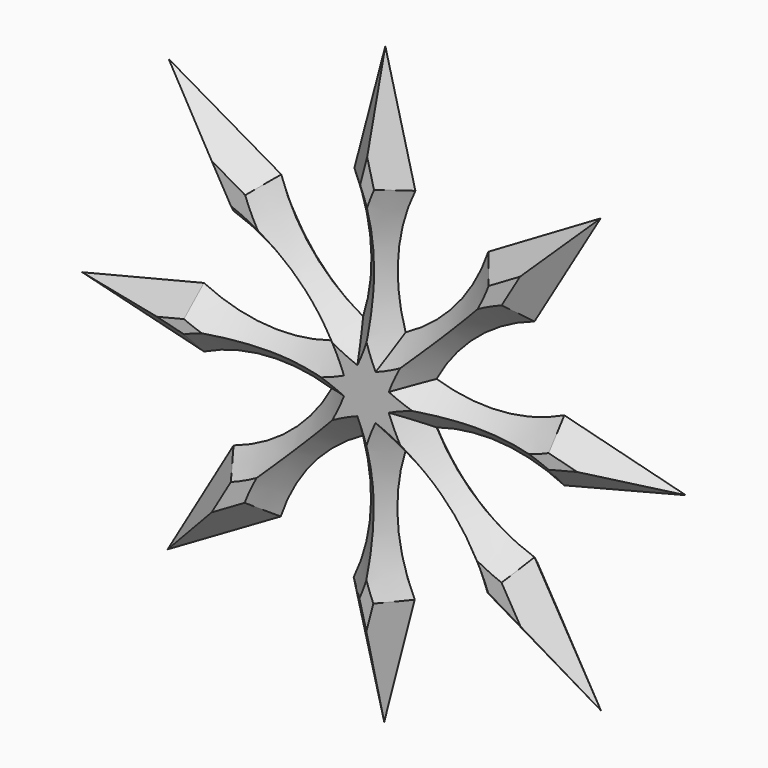
from build123d import *

# Parameters (mm, degrees)
F1_DEPTH      = 3.81
F2_T3_ANGLE   = 94.2071978341
F2_S4_R       = 28.267340588
F2_T5_DEPTH   = 27
F2_T8_DEPTH   = 53.0413211694
F2_T11_DEPTH  = 53.0413211694
F2_T14_ANGLE  = 94.2071978341
F2_S15_R      = 28.267340588
F2_T16_DEPTH  = 27
F2_T19_ANGLE  = 94.2071978341
F2_S20_R      = 28.267340588
F2_T21_DEPTH  = 26
F2_T24_DEPTH  = 53.791822705
F2_T27_DEPTH  = 53.791822705
F2_T30_ANGLE  = 94.2071978341
F2_S31_R      = 28.267340588
F2_T32_DEPTH  = 26
F2_T35_ANGLE  = 94.2071978341
F2_S36_R      = 28.267340588
F2_T37_DEPTH  = 27
F2_T40_DEPTH  = 52.2617558208
F2_T43_DEPTH  = 52.2617558208
F2_T46_ANGLE  = 94.2071978341
F2_S47_R      = 28.267340588
F2_T48_DEPTH  = 27
F2_T51_ANGLE  = 94.2071978341
F2_S52_R      = 28.267340588
F2_T53_DEPTH  = 26
F2_T56_DEPTH  = 53.6108831217
F2_T59_DEPTH  = 53.6108831217
F2_T62_ANGLE  = 94.2071978341
F2_S63_R      = 28.267340588
F2_T64_DEPTH  = 26
F2_T67_ANGLE  = 94.2071978341
F2_S68_R      = 28.267340588
F2_T69_DEPTH  = 27
F2_T72_DEPTH  = 53.1727745631
F2_T75_DEPTH  = 53.1727745631
F2_T78_ANGLE  = 94.2071978341
F2_S79_R      = 28.267340588
F2_T80_DEPTH  = 27
F2_T83_ANGLE  = 94.2071978341
F2_S84_R      = 28.267340588
F2_T85_DEPTH  = 26
F2_T88_DEPTH  = 53.7976919269
F2_T91_DEPTH  = 53.7976919269
F2_T94_ANGLE  = 94.2071978341
F2_S95_R      = 28.267340588
F2_T96_DEPTH  = 26
F2_T99_ANGLE  = 94.2071978341
F2_S100_R     = 28.267340588
F2_T101_DEPTH = 27
F2_T104_DEPTH = 52.2617558208
F2_T107_DEPTH = 52.2617558208
F2_T110_ANGLE = 94.2071978341
F2_S111_R     = 28.267340588
F2_T112_DEPTH = 27
F2_T115_ANGLE = 94.2071978341
F2_S116_R     = 28.267340588
F2_T117_DEPTH = 26
F2_T120_DEPTH = 53.9557904265
F2_T123_DEPTH = 53.9557904265
F2_T126_ANGLE = 94.2071978341
F2_S127_R     = 28.267340588
F2_T128_DEPTH = 26
F2_T132_ANGLE = 94.2071978341
F2_S133_R     = 28.267340588
F2_T134_DEPTH = 27
F2_T138_ANGLE = 94.2071978341
F2_S139_R     = 28.267340588
F2_T140_DEPTH = 26
F2_T146_ANGLE = 94.2071978341
F2_S147_R     = 28.267340588
F2_T148_DEPTH = 27
F2_T152_ANGLE = 94.2071978341
F2_S153_R     = 28.267340588
F2_T154_DEPTH = 26
F2_T160_ANGLE = 94.2071978341
F2_S161_R     = 28.267340588
F2_T162_DEPTH = 26
F2_T166_ANGLE = 94.2071978341
F2_S167_R     = 28.267340588
F2_T168_DEPTH = 27
F2_T174_ANGLE = 94.2071978341
F2_S175_R     = 28.267340588
F2_T176_DEPTH = 27
F2_T180_ANGLE = 94.2071978341
F2_S181_R     = 28.267340588
F2_T182_DEPTH = 26
F2_T188_ANGLE = 94.2071978341
F2_S189_R     = 28.267340588
F2_T190_DEPTH = 26
F2_T194_ANGLE = 94.2071978341
F2_S195_R     = 28.267340588
F2_T196_DEPTH = 27
F2_T202_ANGLE = 94.2071978341
F2_S203_R     = 28.267340588
F2_T204_DEPTH = 27
F2_T208_ANGLE = 94.2071978341
F2_S209_R     = 28.267340588
F2_T210_DEPTH = 26
F2_T216_ANGLE = 94.2071978341
F2_S217_R     = 28.267340588
F2_T218_DEPTH = 26
F2_T222_ANGLE = 94.2071978341
F2_S223_R     = 28.267340588
F2_T224_DEPTH = 27
F2_T230_ANGLE = 94.2071978341
F2_S231_R     = 28.267340588
F2_T232_DEPTH = 27
F2_T236_ANGLE = 94.2071978341
F2_S237_R     = 28.267340588
F2_T238_DEPTH = 26


# Not quite as in the source:
# - a fillet or chamfer that OpenCascade refuses, or shapes differently, is made with other operations: its cross-section is extruded or revolved along the edge and cut away or added


with BuildPart() as f1:
    # F0 (on Front) → F1 (new body)
    with BuildSketch(Plane.XZ):
        with BuildLine():
            Line((6.679601036, 30.6390393525), (0.209001727, 55.9587727979))
            Line((0.209001727, 55.9587727979), (-6.4505489481, 30.6880794563))
            ThreePointArc((-6.4505489481, 30.6880794563), (-3.6066981966, 20.9770503759), (-4.3651827706, 10.8866453272))
            ThreePointArc((-4.3651827706, 10.8866453272), (-11.8846232574, 17.6578776863), (-16.5375233069, 26.6435381532))
            Line((-16.5375233069, 26.6435381532), (-40.327632255, 40.403012619))
            Line((-40.327632255, 40.403012619), (-26.6126086657, 16.5872499967))
            ThreePointArc((-26.6126086657, 16.5872499967), (-17.6356529341, 11.9175777716), (-10.8784745754, 4.3855054456))
            ThreePointArc((-10.8784745754, 4.3855054456), (-20.970278463, 3.6458655403), (-30.6759798559, 6.5078462128))
            Line((-30.6759798559, 6.5078462128), (-56.9257720003, 0))
            Line((-56.9257720003, 0), (-30.6759798559, -6.5078462128))
            ThreePointArc((-30.6759798559, -6.5078462128), (-20.970278463, -3.6458655403), (-10.8784745754, -4.3855054456))
            ThreePointArc((-10.8784745754, -4.3855054456), (-17.6356529341, -11.9175777716), (-26.6126086657, -16.5872499967))
            Line((-26.6126086657, -16.5872499967), (-40.5599377533, -40.4842646123))
            Line((-40.5599377533, -40.4842646123), (-16.6369188404, -26.58158637))
            ThreePointArc((-16.6369188404, -26.58158637), (-11.9504907247, -17.6133666797), (-4.4058128267, -10.8702658862))
            ThreePointArc((-4.4058128267, -10.8702658862), (-3.6850201695, -20.9634334188), (-6.5651207822, -30.6637732767))
            Line((-6.5651207822, -30.6637732767), (0, -55.9591630992))
            Line((0, -55.9591630992), (6.5651207822, -30.6637732767))
            ThreePointArc((6.5651207822, -30.6637732767), (3.6850201695, -20.9634334188), (4.4058128267, -10.8702658862))
            ThreePointArc((4.4058128267, -10.8702658862), (11.9504907247, -17.6133666797), (16.6369188404, -26.58158637))
            Line((16.6369188404, -26.58158637), (40.6195603878, -40.6954864235))
            Line((40.6195603878, -40.6954864235), (26.5504713741, -16.6865296649))
            ThreePointArc((26.5504713741, -16.6865296649), (17.5910190008, -11.9833620019), (10.8620192883, -4.4261048431))
            ThreePointArc((10.8620192883, -4.4261048431), (20.9565152672, -3.7241619477), (30.6514597612, -6.6223724565))
            Line((30.6514597612, -6.6223724565), (56.7369909394, 0))
            Line((56.7369909394, 0), (30.6514597612, 6.6223724565))
            ThreePointArc((30.6514597612, 6.6223724565), (20.9565152672, 3.7241619477), (10.8620192883, 4.4261048431))
            ThreePointArc((10.8620192883, 4.4261048431), (17.5910190008, 11.9833620019), (26.5504713741, 16.6865296649))
            Line((26.5504713741, 16.6865296649), (40.5952992978, 40.5195601823))
            Line((40.5952992978, 40.5195601823), (16.7360822971, 26.5192637868))
            ThreePointArc((16.7360822971, 26.5192637868), (12.0161914886, 17.5686099753), (4.4463814239, 10.8537348104))
            ThreePointArc((4.4463814239, 10.8537348104), (3.7632907382, 20.9495240322), (6.679601036, 30.6390393525))
        make_face()
    extrude(amount=F1_DEPTH)

    # F2: chamfer of 5.08 on 32 edges, made by hand


with BuildPart() as f2_tool1:
    # F2_s2 → F2_t3 (revolve)
    with BuildSketch(Plane(origin=(-5.5052343912, 0, -4.7470845502), x_dir=(0, 1, 0), z_dir=(-0.757328805, 0, -0.6530337519))):
        Polygon((1.27, 7.4792542612), (-3.81, 2.3992542612), (-3.81, 7.4792542612), align=None)
    revolve(axis=Axis((17.838498561, -3.81, -31.8190105099), (0, 1, 0)), revolution_arc=F2_T3_ANGLE)

    # F2_s4 → F2_t5 (intersect, symmetric)
    with BuildSketch(Plane.XZ.offset(1.3)):
        with Locations((34.9970077729, 10.289358954)):
            Circle(F2_S4_R)
    extrude(amount=F2_T5_DEPTH, both=True, mode=Mode.INTERSECT)


with BuildPart() as f2_tool6:
    # F2_s7 → F2_t8 (new body)
    with BuildSketch(Plane(origin=(14.5536608526, 0, 3.6947594478), x_dir=(0, 1, 0), z_dir=(0.9692531432, 0, 0.2460657318))):
        Polygon((1.27, -13.9610291961), (-3.81, -8.8810291961), (-3.81, -13.9610291961), align=None)
    extrude(amount=F2_T8_DEPTH)


with BuildPart() as f2_tool9:
    # F2_s10 → F2_t11 (new body)
    with BuildSketch(Plane(origin=(65.9641281162, 0, -16.7464109574), x_dir=(0, 1, 0), z_dir=(-0.9692531432, 0, 0.2460657318))):
        Polygon((1.27, -13.9610291961), (-3.81, -8.8810291961), (-3.81, -13.9610291961), align=None)
    extrude(amount=F2_T11_DEPTH)


with BuildPart() as f2_tool12:
    # F2_s13 → F2_t14 (revolve)
    with BuildSketch(Plane(origin=(21.55504735, 0, 29.0625266695), x_dir=(0, 1, 0), z_dir=(0.595713721, 0, 0.8031968393))):
        Polygon((1.27, -23.6401451022), (-3.81, -28.7201451022), (-3.81, -23.6401451022), align=None)
    revolve(axis=Axis((17.838498561, -3.81, 31.8190105099), (0, 1, 0)), revolution_arc=F2_T14_ANGLE)

    # F2_s15 → F2_t16 (intersect, symmetric)
    with BuildSketch(Plane.XZ.offset(1.3)):
        with Locations((34.9970077729, -10.289358954)):
            Circle(F2_S15_R)
    extrude(amount=F2_T16_DEPTH, both=True, mode=Mode.INTERSECT)


with BuildPart() as f2_tool17:
    # F2_s18 → F2_t19 (revolve)
    with BuildSketch(Plane(origin=(-0.6195292674, 0, -7.2428310015), x_dir=(0, 1, 0), z_dir=(-0.0852256828, 0, -0.9963616728))):
        Polygon((1.27, 7.4792542612), (-3.81, 2.3992542612), (-3.81, 7.4792542612), align=None)
    revolve(axis=Axis((34.9970077729, -3.81, -10.289358954), (0, 1, 0)), revolution_arc=F2_T19_ANGLE)

    # F2_s20 → F2_t21 (intersect, symmetric)
    with BuildSketch(Plane.XZ.offset(1.3)):
        with Locations((17.838498561, 31.8190105099)):
            Circle(F2_S20_R)
    extrude(amount=F2_T21_DEPTH, both=True, mode=Mode.INTERSECT)


with BuildPart() as f2_tool22:
    # F2_s23 → F2_t24 (new body)
    with BuildSketch(Plane(origin=(7.5097109066, 0, 12.7434220047), x_dir=(0, 1, 0), z_dir=(0.5077020612, 0, 0.8615327139))):
        Polygon((1.27, -14.4023141537), (-3.81, -9.3223141537), (-3.81, -14.4023141537), align=None)
    extrude(amount=F2_T24_DEPTH)


with BuildPart() as f2_tool25:
    # F2_s26 → F2_t27 (new body)
    with BuildSketch(Plane(origin=(59.1517585206, 0, 34.7095276255), x_dir=(0, 1, 0), z_dir=(-0.8624793208, 0, -0.506092305))):
        Polygon((1.27, -14.4023141537), (-3.81, -9.3223141537), (-3.81, -14.4023141537), align=None)
    extrude(amount=F2_T27_DEPTH)


with BuildPart() as f2_tool28:
    # F2_s29 → F2_t30 (revolve)
    with BuildSketch(Plane(origin=(-5.6536224324, 0, 35.7391532646), x_dir=(0, 1, 0), z_dir=(-0.1562483441, 0, 0.9877178013))):
        Polygon((1.27, -23.6401451022), (-3.81, -28.7201451022), (-3.81, -23.6401451022), align=None)
    revolve(axis=Axis((-10.2239857837, -3.81, 35.0161616319), (0, 1, 0)), revolution_arc=F2_T30_ANGLE)

    # F2_s31 → F2_t32 (intersect, symmetric)
    with BuildSketch(Plane.XZ.offset(1.3)):
        with Locations((31.8522675655, 17.7790469844)):
            Circle(F2_S31_R)
    extrude(amount=F2_T32_DEPTH, both=True, mode=Mode.INTERSECT)


with BuildPart() as f2_tool33:
    # F2_s34 → F2_t35 (revolve)
    with BuildSketch(Plane(origin=(4.7367955124, 0, -5.5140897439), x_dir=(0, 1, 0), z_dir=(0.6516183381, 0, -0.7585469936))):
        Polygon((1.27, 7.4792542612), (-3.81, 2.3992542612), (-3.81, 7.4792542612), align=None)
    revolve(axis=Axis((31.8522675655, -3.81, 17.7790469844), (0, 1, 0)), revolution_arc=F2_T35_ANGLE)

    # F2_s36 → F2_t37 (intersect, symmetric)
    with BuildSketch(Plane.XZ.offset(1.3)):
        with Locations((-10.2239857837, 35.0161616319)):
            Circle(F2_S36_R)
    extrude(amount=F2_T37_DEPTH, both=True, mode=Mode.INTERSECT)


with BuildPart() as f2_tool38:
    # F2_s39 → F2_t40 (new body)
    with BuildSketch(Plane(origin=(-3.7058079888, 0, 14.5009860748), x_dir=(0, 1, 0), z_dir=(-0.2475982949, 0, 0.9688627789))):
        Polygon((1.27, -14.0577907221), (-3.81, -8.9777907221), (-3.81, -14.0577907221), align=None)
    extrude(amount=F2_T40_DEPTH)


with BuildPart() as f2_tool41:
    # F2_s42 → F2_t43 (new body)
    with BuildSketch(Plane(origin=(17.1318103034, 0, 65.0092995281), x_dir=(0, 1, 0), z_dir=(-0.2548285426, 0, -0.9669862532))):
        Polygon((1.27, -14.0577907221), (-3.81, -8.9777907221), (-3.81, -14.0577907221), align=None)
    extrude(amount=F2_T43_DEPTH)


with BuildPart() as f2_tool44:
    # F2_s45 → F2_t46 (revolve)
    with BuildSketch(Plane(origin=(-28.9413121051, 0, 21.7175269383), x_dir=(0, 1, 0), z_dir=(-0.7998468499, 0, 0.6002041458))):
        Polygon((1.27, -23.6401451022), (-3.81, -28.7201451022), (-3.81, -23.6401451022), align=None)
    revolve(axis=Axis((-31.718574019, -3.81, 18.0164792049), (0, 1, 0)), revolution_arc=F2_T46_ANGLE)

    # F2_s47 → F2_t48 (intersect, symmetric)
    with BuildSketch(Plane.XZ.offset(1.3)):
        with Locations((10.4852622562, 34.9388141779)):
            Circle(F2_S47_R)
    extrude(amount=F2_T48_DEPTH, both=True, mode=Mode.INTERSECT)


with BuildPart() as f2_tool49:
    # F2_s50 → F2_t51 (revolve)
    with BuildSketch(Plane(origin=(7.2392465313, 0, -0.660096272), x_dir=(0, 1, 0), z_dir=(0.9958685743, 0, -0.0908062919))):
        Polygon((1.27, 7.4792542612), (-3.81, 2.3992542612), (-3.81, 7.4792542612), align=None)
    revolve(axis=Axis((10.4852622562, -3.81, 34.9388141779), (0, 1, 0)), revolution_arc=F2_T51_ANGLE)

    # F2_s52 → F2_t53 (intersect, symmetric)
    with BuildSketch(Plane.XZ.offset(1.3)):
        with Locations((-31.718574019, 18.0164792049)):
            Circle(F2_S52_R)
    extrude(amount=F2_T53_DEPTH, both=True, mode=Mode.INTERSECT)


with BuildPart() as f2_tool54:
    # F2_s55 → F2_t56 (new body)
    with BuildSketch(Plane(origin=(-12.6304595626, 0, 7.3050731387), x_dir=(0, 1, 0), z_dir=(-0.8656430916, 0, 0.5006616002))):
        Polygon((1.27, -14.7840918558), (-3.81, -9.7040918558), (-3.81, -14.7840918558), align=None)
    extrude(amount=F2_T56_DEPTH)


with BuildPart() as f2_tool57:
    # F2_s58 → F2_t59 (new body)
    with BuildSketch(Plane(origin=(-34.0356728526, 0, 59.1020132098), x_dir=(0, 1, 0), z_dir=(0.4990441804, 0, -0.8665765437))):
        Polygon((1.27, -14.7840918558), (-3.81, -9.7040918558), (-3.81, -14.7840918558), align=None)
    extrude(amount=F2_T59_DEPTH)


with BuildPart() as f2_tool60:
    # F2_s61 → F2_t62 (revolve)
    with BuildSketch(Plane(origin=(-35.7069189472, 0, -5.8537562277), x_dir=(0, 1, 0), z_dir=(-0.9868269461, 0, -0.1617794128))):
        Polygon((1.27, -23.6401451022), (-3.81, -28.7201451022), (-3.81, -23.6401451022), align=None)
    revolve(axis=Axis((-34.9583339784, -3.81, -10.419997418), (0, 1, 0)), revolution_arc=F2_T62_ANGLE)

    # F2_s63 → F2_t64 (intersect, symmetric)
    with BuildSketch(Plane.XZ.offset(1.3)):
        with Locations((-17.9572148782, 31.7521636201)):
            Circle(F2_S63_R)
    extrude(amount=F2_T64_DEPTH, both=True, mode=Mode.INTERSECT)


with BuildPart() as f2_tool65:
    # F2_s66 → F2_t67 (revolve)
    with BuildSketch(Plane(origin=(5.4874661203, 0, 4.7676129256), x_dir=(0, 1, 0), z_dir=(0.7548845088, 0, 0.6558577425))):
        Polygon((1.27, 7.4792542612), (-3.81, 2.3992542612), (-3.81, 7.4792542612), align=None)
    revolve(axis=Axis((-17.9572148782, -3.81, 31.7521636201), (0, 1, 0)), revolution_arc=F2_T67_ANGLE)

    # F2_s68 → F2_t69 (intersect, symmetric)
    with BuildSketch(Plane.XZ.offset(1.3)):
        with Locations((-34.9583339784, -10.419997418)):
            Circle(F2_S68_R)
    extrude(amount=F2_T69_DEPTH, both=True, mode=Mode.INTERSECT)


with BuildPart() as f2_tool70:
    # F2_s71 → F2_t72 (new body)
    with BuildSketch(Plane(origin=(-14.6994140485, 0, -3.6442774678), x_dir=(0, 1, 0), z_dir=(-0.9706156896, 0, -0.2406349584))):
        Polygon((1.27, -13.6983307744), (-3.81, -8.6183307744), (-3.81, -13.6983307744), align=None)
    extrude(amount=F2_T72_DEPTH)


with BuildPart() as f2_tool73:
    # F2_s74 → F2_t75 (new body)
    with BuildSketch(Plane(origin=(-66.3097432969, 0, 16.4395058602), x_dir=(0, 1, 0), z_dir=(0.9706156896, 0, -0.2406349584))):
        Polygon((1.27, -13.6983307744), (-3.81, -8.6183307744), (-3.81, -13.6983307744), align=None)
    extrude(amount=F2_T75_DEPTH)


with BuildPart() as f2_tool76:
    # F2_s77 → F2_t78 (revolve)
    with BuildSketch(Plane(origin=(-21.6634425612, 0, -28.9818180774), x_dir=(0, 1, 0), z_dir=(-0.5987094237, 0, -0.8009663076))):
        Polygon((1.27, -23.6401451022), (-3.81, -28.7201451022), (-3.81, -23.6401451022), align=None)
    revolve(axis=Axis((-17.9572148782, -3.81, -31.7521636201), (0, 1, 0)), revolution_arc=F2_T78_ANGLE)

    # F2_s79 → F2_t80 (intersect, symmetric)
    with BuildSketch(Plane.XZ.offset(1.3)):
        with Locations((-34.9583339784, 10.419997418)):
            Circle(F2_S79_R)
    extrude(amount=F2_T80_DEPTH, both=True, mode=Mode.INTERSECT)


with BuildPart() as f2_tool81:
    # F2_s82 → F2_t83 (revolve)
    with BuildSketch(Plane(origin=(0.6465761763, 0, 7.2404666064), x_dir=(0, 1, 0), z_dir=(0.0889463969, 0, 0.9960364142))):
        Polygon((1.27, 7.4792542612), (-3.81, 2.3992542612), (-3.81, 7.4792542612), align=None)
    revolve(axis=Axis((-34.9583339784, -3.81, 10.419997418), (0, 1, 0)), revolution_arc=F2_T83_ANGLE)

    # F2_s84 → F2_t85 (intersect, symmetric)
    with BuildSketch(Plane.XZ.offset(1.3)):
        with Locations((-17.9572148782, -31.7521636201)):
            Circle(F2_S84_R)
    extrude(amount=F2_T85_DEPTH, both=True, mode=Mode.INTERSECT)


with BuildPart() as f2_tool86:
    # F2_s87 → F2_t88 (new body)
    with BuildSketch(Plane(origin=(-7.3978771417, 0, -12.6753428609), x_dir=(0, 1, 0), z_dir=(-0.5040706605, 0, -0.8636624163))):
        Polygon((1.27, -14.6231638423), (-3.81, -9.5431638423), (-3.81, -14.6231638423), align=None)
    extrude(amount=F2_T88_DEPTH)


with BuildPart() as f2_tool89:
    # F2_s90 → F2_t91 (new body)
    with BuildSketch(Plane(origin=(-59.2027407791, 0, -34.4052169633), x_dir=(0, 1, 0), z_dir=(0.864602238, 0, 0.5024569335))):
        Polygon((1.27, -14.6231638423), (-3.81, -9.5431638423), (-3.81, -14.6231638423), align=None)
    extrude(amount=F2_T91_DEPTH)


with BuildPart() as f2_tool92:
    # F2_s93 → F2_t94 (revolve)
    with BuildSketch(Plane(origin=(5.7870650668, 0, -35.7177882936), x_dir=(0, 1, 0), z_dir=(0.1599362789, 0, -0.9871273407))):
        Polygon((1.27, -23.6401451022), (-3.81, -28.7201451022), (-3.81, -23.6401451022), align=None)
    revolve(axis=Axis((10.3546962414, -3.81, -34.977731866), (0, 1, 0)), revolution_arc=F2_T94_ANGLE)

    # F2_s95 → F2_t96 (intersect, symmetric)
    with BuildSketch(Plane.XZ.offset(1.3)):
        with Locations((-31.7856424893, -17.897887928)):
            Circle(F2_S95_R)
    extrude(amount=F2_T96_DEPTH, both=True, mode=Mode.INTERSECT)


with BuildPart() as f2_tool97:
    # F2_s98 → F2_t99 (revolve)
    with BuildSketch(Plane(origin=(-4.7573570333, 0, 5.4963598397), x_dir=(0, 1, 0), z_dir=(-0.6544468883, 0, 0.7561079753))):
        Polygon((1.27, 7.4792542612), (-3.81, 2.3992542612), (-3.81, 7.4792542612), align=None)
    revolve(axis=Axis((-31.7856424893, -3.81, -17.897887928), (0, 1, 0)), revolution_arc=F2_T99_ANGLE)

    # F2_s100 → F2_t101 (intersect, symmetric)
    with BuildSketch(Plane.XZ.offset(1.3)):
        with Locations((10.3546962414, -34.977731866)):
            Circle(F2_S100_R)
    extrude(amount=F2_T101_DEPTH, both=True, mode=Mode.INTERSECT)


with BuildPart() as f2_tool102:
    # F2_s103 → F2_t104 (new body)
    with BuildSketch(Plane(origin=(3.7599418354, 0, -14.4870441218), x_dir=(0, 1, 0), z_dir=(0.2512151709, 0, -0.9679312671))):
        Polygon((1.27, -14.0577907221), (-3.81, -8.9777907221), (-3.81, -14.0577907221), align=None)
    extrude(amount=F2_T104_DEPTH)


with BuildPart() as f2_tool105:
    # F2_s106 → F2_t107 (new body)
    with BuildSketch(Plane(origin=(-16.8888877561, 0, -65.0728316563), x_dir=(0, 1, 0), z_dir=(0.2512151709, 0, 0.9679312671))):
        Polygon((1.27, -14.0577907221), (-3.81, -8.9777907221), (-3.81, -14.0577907221), align=None)
    extrude(amount=F2_T107_DEPTH)


with BuildPart() as f2_tool108:
    # F2_s109 → F2_t110 (revolve)
    with BuildSketch(Plane(origin=(29.0222229792, 0, -21.6092826355), x_dir=(0, 1, 0), z_dir=(0.8020829721, 0, -0.5972126137))):
        Polygon((1.27, -23.6401451022), (-3.81, -28.7201451022), (-3.81, -23.6401451022), align=None)
    revolve(axis=Axis((31.7856424893, -3.81, -17.897887928), (0, 1, 0)), revolution_arc=F2_T110_ANGLE)

    # F2_s111 → F2_t112 (intersect, symmetric)
    with BuildSketch(Plane.XZ.offset(1.3)):
        with Locations((-10.3546962414, -34.977731866)):
            Circle(F2_S111_R)
    extrude(amount=F2_T112_DEPTH, both=True, mode=Mode.INTERSECT)


with BuildPart() as f2_tool113:
    # F2_s114 → F2_t115 (revolve)
    with BuildSketch(Plane(origin=(-7.2416614312, 0, 0.6330538257), x_dir=(0, 1, 0), z_dir=(-0.9962007806, 0, 0.0870861917))):
        Polygon((1.27, 7.4792542612), (-3.81, 2.3992542612), (-3.81, 7.4792542612), align=None)
    revolve(axis=Axis((-10.3546962414, -3.81, -34.977731866), (0, 1, 0)), revolution_arc=F2_T115_ANGLE)

    # F2_s116 → F2_t117 (intersect, symmetric)
    with BuildSketch(Plane.XZ.offset(1.3)):
        with Locations((31.7856424893, -17.897887928)):
            Circle(F2_S116_R)
    extrude(amount=F2_T117_DEPTH, both=True, mode=Mode.INTERSECT)


with BuildPart() as f2_tool118:
    # F2_s119 → F2_t120 (new body)
    with BuildSketch(Plane(origin=(12.7172695414, 0, -7.4841743728), x_dir=(0, 1, 0), z_dir=(0.8618326861, 0, -0.5071926864))):
        Polygon((1.27, -14.4707564211), (-3.81, -9.3907564211), (-3.81, -14.4707564211), align=None)
    extrude(amount=F2_T120_DEPTH)


with BuildPart() as f2_tool121:
    # F2_s122 → F2_t123 (new body)
    with BuildSketch(Plane(origin=(34.7395088846, 0, -59.2831110683), x_dir=(0, 1, 0), z_dir=(-0.505582371, 0, 0.8627783413))):
        Polygon((1.27, -14.4707564211), (-3.81, -9.3907564211), (-3.81, -14.4707564211), align=None)
    extrude(amount=F2_T123_DEPTH)


with BuildPart() as f2_tool124:
    # F2_s125 → F2_t126 (revolve)
    with BuildSketch(Plane(origin=(35.7285330786, 0, 5.7203537241), x_dir=(0, 1, 0), z_dir=(0.9874242927, 0, 0.1580925872))):
        Polygon((1.27, -23.6401451022), (-3.81, -28.7201451022), (-3.81, -23.6401451022), align=None)
    revolve(axis=Axis((34.9970077729, -3.81, 10.289358954), (0, 1, 0)), revolution_arc=F2_T126_ANGLE)

    # F2_s127 → F2_t128 (intersect, symmetric)
    with BuildSketch(Plane.XZ.offset(1.3)):
        with Locations((17.838498561, -31.8190105099)):
            Circle(F2_S127_R)
    extrude(amount=F2_T128_DEPTH, both=True, mode=Mode.INTERSECT)


with BuildPart() as f2_tool130:
    # F2_s131 → F2_t132 (revolve)
    with BuildSketch(Plane(origin=(-5.5052343912, 0, -4.7470845502), x_dir=(0, 1, 0), z_dir=(-0.757328805, 0, -0.6530337519))):
        Polygon((1.27, 7.4792542612), (-3.81, 2.3992542612), (-3.81, 7.4792542612), align=None)
    revolve(axis=Axis((17.838498561, -3.81, -31.8190105099), (0, 1, 0)), revolution_arc=F2_T132_ANGLE)

    # F2_s133 → F2_t134 (cut, symmetric)
    with BuildSketch(Plane.XZ.offset(1.3)):
        with Locations((34.9970077729, 10.289358954)):
            Circle(F2_S133_R)
    extrude(amount=F2_T134_DEPTH, both=True, mode=Mode.SUBTRACT)

    split(bisect_by=Plane.XZ, keep=Keep.TOP)


with BuildPart() as f2_tool136:
    # F2_s137 → F2_t138 (revolve)
    with BuildSketch(Plane(origin=(35.7285330786, 0, 5.7203537241), x_dir=(0, 1, 0), z_dir=(0.9874242927, 0, 0.1580925872))):
        Polygon((1.27, -23.6401451022), (-3.81, -28.7201451022), (-3.81, -23.6401451022), align=None)
    revolve(axis=Axis((34.9970077729, -3.81, 10.289358954), (0, 1, 0)), revolution_arc=F2_T138_ANGLE)

    # F2_s139 → F2_t140 (cut, symmetric)
    with BuildSketch(Plane.XZ.offset(1.3)):
        with Locations((17.838498561, -31.8190105099)):
            Circle(F2_S139_R)
    extrude(amount=F2_T140_DEPTH, both=True, mode=Mode.SUBTRACT)

    split(bisect_by=Plane.XZ, keep=Keep.TOP)


with BuildPart() as f2_tool130_1:
    add(f2_tool130.part)

    # F2_t142: intersect F2_tool136
    add(f2_tool136.part, mode=Mode.INTERSECT)


with BuildPart() as f2_tool144:
    # F2_s145 → F2_t146 (revolve)
    with BuildSketch(Plane(origin=(21.55504735, 0, 29.0625266695), x_dir=(0, 1, 0), z_dir=(0.595713721, 0, 0.8031968393))):
        Polygon((1.27, -23.6401451022), (-3.81, -28.7201451022), (-3.81, -23.6401451022), align=None)
    revolve(axis=Axis((17.838498561, -3.81, 31.8190105099), (0, 1, 0)), revolution_arc=F2_T146_ANGLE)

    # F2_s147 → F2_t148 (cut, symmetric)
    with BuildSketch(Plane.XZ.offset(1.3)):
        with Locations((34.9970077729, -10.289358954)):
            Circle(F2_S147_R)
    extrude(amount=F2_T148_DEPTH, both=True, mode=Mode.SUBTRACT)

    split(bisect_by=Plane.XZ, keep=Keep.TOP)


with BuildPart() as f2_tool150:
    # F2_s151 → F2_t152 (revolve)
    with BuildSketch(Plane(origin=(-0.6195292674, 0, -7.2428310015), x_dir=(0, 1, 0), z_dir=(-0.0852256828, 0, -0.9963616728))):
        Polygon((1.27, 7.4792542612), (-3.81, 2.3992542612), (-3.81, 7.4792542612), align=None)
    revolve(axis=Axis((34.9970077729, -3.81, -10.289358954), (0, 1, 0)), revolution_arc=F2_T152_ANGLE)

    # F2_s153 → F2_t154 (cut, symmetric)
    with BuildSketch(Plane.XZ.offset(1.3)):
        with Locations((17.838498561, 31.8190105099)):
            Circle(F2_S153_R)
    extrude(amount=F2_T154_DEPTH, both=True, mode=Mode.SUBTRACT)

    split(bisect_by=Plane.XZ, keep=Keep.TOP)


with BuildPart() as f2_tool144_1:
    add(f2_tool144.part)

    # F2_t156: intersect F2_tool150
    add(f2_tool150.part, mode=Mode.INTERSECT)


with BuildPart() as f2_tool158:
    # F2_s159 → F2_t160 (revolve)
    with BuildSketch(Plane(origin=(-5.6536224324, 0, 35.7391532646), x_dir=(0, 1, 0), z_dir=(-0.1562483441, 0, 0.9877178013))):
        Polygon((1.27, -23.6401451022), (-3.81, -28.7201451022), (-3.81, -23.6401451022), align=None)
    revolve(axis=Axis((-10.2239857837, -3.81, 35.0161616319), (0, 1, 0)), revolution_arc=F2_T160_ANGLE)

    # F2_s161 → F2_t162 (cut, symmetric)
    with BuildSketch(Plane.XZ.offset(1.3)):
        with Locations((31.8522675655, 17.7790469844)):
            Circle(F2_S161_R)
    extrude(amount=F2_T162_DEPTH, both=True, mode=Mode.SUBTRACT)

    split(bisect_by=Plane.XZ, keep=Keep.TOP)


with BuildPart() as f2_tool164:
    # F2_s165 → F2_t166 (revolve)
    with BuildSketch(Plane(origin=(4.7367955124, 0, -5.5140897439), x_dir=(0, 1, 0), z_dir=(0.6516183381, 0, -0.7585469936))):
        Polygon((1.27, 7.4792542612), (-3.81, 2.3992542612), (-3.81, 7.4792542612), align=None)
    revolve(axis=Axis((31.8522675655, -3.81, 17.7790469844), (0, 1, 0)), revolution_arc=F2_T166_ANGLE)

    # F2_s167 → F2_t168 (cut, symmetric)
    with BuildSketch(Plane.XZ.offset(1.3)):
        with Locations((-10.2239857837, 35.0161616319)):
            Circle(F2_S167_R)
    extrude(amount=F2_T168_DEPTH, both=True, mode=Mode.SUBTRACT)

    split(bisect_by=Plane.XZ, keep=Keep.TOP)


with BuildPart() as f2_tool158_1:
    add(f2_tool158.part)

    # F2_t170: intersect F2_tool164
    add(f2_tool164.part, mode=Mode.INTERSECT)


with BuildPart() as f2_tool172:
    # F2_s173 → F2_t174 (revolve)
    with BuildSketch(Plane(origin=(-28.9413121051, 0, 21.7175269383), x_dir=(0, 1, 0), z_dir=(-0.7998468499, 0, 0.6002041458))):
        Polygon((1.27, -23.6401451022), (-3.81, -28.7201451022), (-3.81, -23.6401451022), align=None)
    revolve(axis=Axis((-31.718574019, -3.81, 18.0164792049), (0, 1, 0)), revolution_arc=F2_T174_ANGLE)

    # F2_s175 → F2_t176 (cut, symmetric)
    with BuildSketch(Plane.XZ.offset(1.3)):
        with Locations((10.4852622562, 34.9388141779)):
            Circle(F2_S175_R)
    extrude(amount=F2_T176_DEPTH, both=True, mode=Mode.SUBTRACT)

    split(bisect_by=Plane.XZ, keep=Keep.TOP)


with BuildPart() as f2_tool178:
    # F2_s179 → F2_t180 (revolve)
    with BuildSketch(Plane(origin=(7.2392465313, 0, -0.660096272), x_dir=(0, 1, 0), z_dir=(0.9958685743, 0, -0.0908062919))):
        Polygon((1.27, 7.4792542612), (-3.81, 2.3992542612), (-3.81, 7.4792542612), align=None)
    revolve(axis=Axis((10.4852622562, -3.81, 34.9388141779), (0, 1, 0)), revolution_arc=F2_T180_ANGLE)

    # F2_s181 → F2_t182 (cut, symmetric)
    with BuildSketch(Plane.XZ.offset(1.3)):
        with Locations((-31.718574019, 18.0164792049)):
            Circle(F2_S181_R)
    extrude(amount=F2_T182_DEPTH, both=True, mode=Mode.SUBTRACT)

    split(bisect_by=Plane.XZ, keep=Keep.TOP)


with BuildPart() as f2_tool172_1:
    add(f2_tool172.part)

    # F2_t184: intersect F2_tool178
    add(f2_tool178.part, mode=Mode.INTERSECT)


with BuildPart() as f2_tool186:
    # F2_s187 → F2_t188 (revolve)
    with BuildSketch(Plane(origin=(-35.7069189472, 0, -5.8537562277), x_dir=(0, 1, 0), z_dir=(-0.9868269461, 0, -0.1617794128))):
        Polygon((1.27, -23.6401451022), (-3.81, -28.7201451022), (-3.81, -23.6401451022), align=None)
    revolve(axis=Axis((-34.9583339784, -3.81, -10.419997418), (0, 1, 0)), revolution_arc=F2_T188_ANGLE)

    # F2_s189 → F2_t190 (cut, symmetric)
    with BuildSketch(Plane.XZ.offset(1.3)):
        with Locations((-17.9572148782, 31.7521636201)):
            Circle(F2_S189_R)
    extrude(amount=F2_T190_DEPTH, both=True, mode=Mode.SUBTRACT)

    split(bisect_by=Plane.XZ, keep=Keep.TOP)


with BuildPart() as f2_tool192:
    # F2_s193 → F2_t194 (revolve)
    with BuildSketch(Plane(origin=(5.4874661203, 0, 4.7676129256), x_dir=(0, 1, 0), z_dir=(0.7548845088, 0, 0.6558577425))):
        Polygon((1.27, 7.4792542612), (-3.81, 2.3992542612), (-3.81, 7.4792542612), align=None)
    revolve(axis=Axis((-17.9572148782, -3.81, 31.7521636201), (0, 1, 0)), revolution_arc=F2_T194_ANGLE)

    # F2_s195 → F2_t196 (cut, symmetric)
    with BuildSketch(Plane.XZ.offset(1.3)):
        with Locations((-34.9583339784, -10.419997418)):
            Circle(F2_S195_R)
    extrude(amount=F2_T196_DEPTH, both=True, mode=Mode.SUBTRACT)

    split(bisect_by=Plane.XZ, keep=Keep.TOP)


with BuildPart() as f2_tool186_1:
    add(f2_tool186.part)

    # F2_t198: intersect F2_tool192
    add(f2_tool192.part, mode=Mode.INTERSECT)


with BuildPart() as f2_tool200:
    # F2_s201 → F2_t202 (revolve)
    with BuildSketch(Plane(origin=(-21.6634425612, 0, -28.9818180774), x_dir=(0, 1, 0), z_dir=(-0.5987094237, 0, -0.8009663076))):
        Polygon((1.27, -23.6401451022), (-3.81, -28.7201451022), (-3.81, -23.6401451022), align=None)
    revolve(axis=Axis((-17.9572148782, -3.81, -31.7521636201), (0, 1, 0)), revolution_arc=F2_T202_ANGLE)

    # F2_s203 → F2_t204 (cut, symmetric)
    with BuildSketch(Plane.XZ.offset(1.3)):
        with Locations((-34.9583339784, 10.419997418)):
            Circle(F2_S203_R)
    extrude(amount=F2_T204_DEPTH, both=True, mode=Mode.SUBTRACT)

    split(bisect_by=Plane.XZ, keep=Keep.TOP)


with BuildPart() as f2_tool206:
    # F2_s207 → F2_t208 (revolve)
    with BuildSketch(Plane(origin=(0.6465761763, 0, 7.2404666064), x_dir=(0, 1, 0), z_dir=(0.0889463969, 0, 0.9960364142))):
        Polygon((1.27, 7.4792542612), (-3.81, 2.3992542612), (-3.81, 7.4792542612), align=None)
    revolve(axis=Axis((-34.9583339784, -3.81, 10.419997418), (0, 1, 0)), revolution_arc=F2_T208_ANGLE)

    # F2_s209 → F2_t210 (cut, symmetric)
    with BuildSketch(Plane.XZ.offset(1.3)):
        with Locations((-17.9572148782, -31.7521636201)):
            Circle(F2_S209_R)
    extrude(amount=F2_T210_DEPTH, both=True, mode=Mode.SUBTRACT)

    split(bisect_by=Plane.XZ, keep=Keep.TOP)


with BuildPart() as f2_tool200_1:
    add(f2_tool200.part)

    # F2_t212: intersect F2_tool206
    add(f2_tool206.part, mode=Mode.INTERSECT)


with BuildPart() as f2_tool214:
    # F2_s215 → F2_t216 (revolve)
    with BuildSketch(Plane(origin=(5.7870650668, 0, -35.7177882936), x_dir=(0, 1, 0), z_dir=(0.1599362789, 0, -0.9871273407))):
        Polygon((1.27, -23.6401451022), (-3.81, -28.7201451022), (-3.81, -23.6401451022), align=None)
    revolve(axis=Axis((10.3546962414, -3.81, -34.977731866), (0, 1, 0)), revolution_arc=F2_T216_ANGLE)

    # F2_s217 → F2_t218 (cut, symmetric)
    with BuildSketch(Plane.XZ.offset(1.3)):
        with Locations((-31.7856424893, -17.897887928)):
            Circle(F2_S217_R)
    extrude(amount=F2_T218_DEPTH, both=True, mode=Mode.SUBTRACT)

    split(bisect_by=Plane.XZ, keep=Keep.TOP)


with BuildPart() as f2_tool220:
    # F2_s221 → F2_t222 (revolve)
    with BuildSketch(Plane(origin=(-4.7573570333, 0, 5.4963598397), x_dir=(0, 1, 0), z_dir=(-0.6544468883, 0, 0.7561079753))):
        Polygon((1.27, 7.4792542612), (-3.81, 2.3992542612), (-3.81, 7.4792542612), align=None)
    revolve(axis=Axis((-31.7856424893, -3.81, -17.897887928), (0, 1, 0)), revolution_arc=F2_T222_ANGLE)

    # F2_s223 → F2_t224 (cut, symmetric)
    with BuildSketch(Plane.XZ.offset(1.3)):
        with Locations((10.3546962414, -34.977731866)):
            Circle(F2_S223_R)
    extrude(amount=F2_T224_DEPTH, both=True, mode=Mode.SUBTRACT)

    split(bisect_by=Plane.XZ, keep=Keep.TOP)


with BuildPart() as f2_tool214_1:
    add(f2_tool214.part)

    # F2_t226: intersect F2_tool220
    add(f2_tool220.part, mode=Mode.INTERSECT)


with BuildPart() as f2_tool228:
    # F2_s229 → F2_t230 (revolve)
    with BuildSketch(Plane(origin=(29.0222229792, 0, -21.6092826355), x_dir=(0, 1, 0), z_dir=(0.8020829721, 0, -0.5972126137))):
        Polygon((1.27, -23.6401451022), (-3.81, -28.7201451022), (-3.81, -23.6401451022), align=None)
    revolve(axis=Axis((31.7856424893, -3.81, -17.897887928), (0, 1, 0)), revolution_arc=F2_T230_ANGLE)

    # F2_s231 → F2_t232 (cut, symmetric)
    with BuildSketch(Plane.XZ.offset(1.3)):
        with Locations((-10.3546962414, -34.977731866)):
            Circle(F2_S231_R)
    extrude(amount=F2_T232_DEPTH, both=True, mode=Mode.SUBTRACT)

    split(bisect_by=Plane.XZ, keep=Keep.TOP)


with BuildPart() as f2_tool234:
    # F2_s235 → F2_t236 (revolve)
    with BuildSketch(Plane(origin=(-7.2416614312, 0, 0.6330538257), x_dir=(0, 1, 0), z_dir=(-0.9962007806, 0, 0.0870861917))):
        Polygon((1.27, 7.4792542612), (-3.81, 2.3992542612), (-3.81, 7.4792542612), align=None)
    revolve(axis=Axis((-10.3546962414, -3.81, -34.977731866), (0, 1, 0)), revolution_arc=F2_T236_ANGLE)

    # F2_s237 → F2_t238 (cut, symmetric)
    with BuildSketch(Plane.XZ.offset(1.3)):
        with Locations((31.7856424893, -17.897887928)):
            Circle(F2_S237_R)
    extrude(amount=F2_T238_DEPTH, both=True, mode=Mode.SUBTRACT)

    split(bisect_by=Plane.XZ, keep=Keep.TOP)


with BuildPart() as f2_tool228_1:
    add(f2_tool228.part)

    # F2_t240: intersect F2_tool234
    add(f2_tool234.part, mode=Mode.INTERSECT)


with BuildPart() as f1_1:
    add(f1.part)

    # F2_t241: cut F2_tool1, F2_tool6, F2_tool9, F2_tool12, F2_tool17, F2_tool22, F2_tool25, F2_tool28, F2_tool33, F2_tool38, F2_tool41, F2_tool44, F2_tool49, F2_tool54, F2_tool57, F2_tool60, F2_tool65, F2_tool70, F2_tool73, F2_tool76, F2_tool81, F2_tool86, F2_tool89, F2_tool92, F2_tool97, F2_tool102, F2_tool105, F2_tool108, F2_tool113, F2_tool118, F2_tool121, F2_tool124, F2_tool130, F2_tool144, F2_tool158, F2_tool172, F2_tool186, F2_tool200, F2_tool214, F2_tool228
    add([f2_tool1.part, f2_tool6.part, f2_tool9.part, f2_tool12.part, f2_tool17.part, f2_tool22.part, f2_tool25.part, f2_tool28.part, f2_tool33.part, f2_tool38.part, f2_tool41.part, f2_tool44.part, f2_tool49.part, f2_tool54.part, f2_tool57.part, f2_tool60.part, f2_tool65.part, f2_tool70.part, f2_tool73.part, f2_tool76.part, f2_tool81.part, f2_tool86.part, f2_tool89.part, f2_tool92.part, f2_tool97.part, f2_tool102.part, f2_tool105.part, f2_tool108.part, f2_tool113.part, f2_tool118.part, f2_tool121.part, f2_tool124.part, f2_tool130_1.part, f2_tool144_1.part, f2_tool158_1.part, f2_tool172_1.part, f2_tool186_1.part, f2_tool200_1.part, f2_tool214_1.part, f2_tool228_1.part], mode=Mode.SUBTRACT)

    # F3: F1 across plane


with BuildPart() as f1_2:
    add(f1_1.part)
    add(f1_1.part.mirror(Plane.XZ))


solid = f1_2.part
